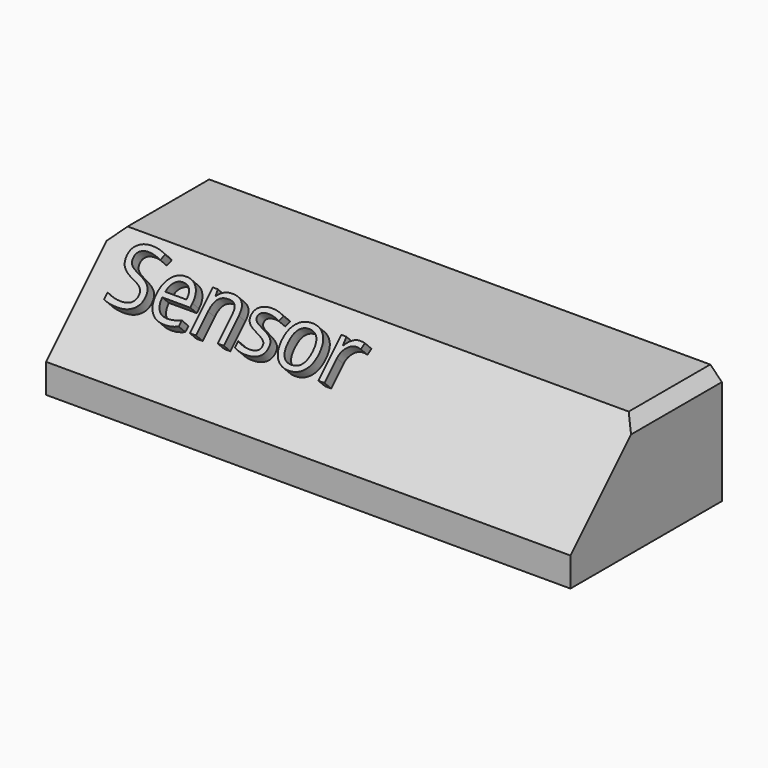
from build123d import *

# Parameters (mm, degrees)
F0_W         = 114.3
F0_H         = 41.275
F1_DEPTH     = 25.4
F2_SIZE      = 19.05
F3_SIZE      = 2.54
F4_TEXT_SIZE = 16.5284106818
F5_DEPTH     = 2.54


# Not quite as in the source:
# - Text() gives the source's letters only with a copy of the font that has no kerning and outlines rounded to 1/6400 em; it was checked with that copy


with BuildPart() as f1:
    # F0 (on Top) → F1 (new body)
    with BuildSketch(Plane.XY):
        with Locations((0, -20.6375)):
            Rectangle(F0_W, F0_H)
    extrude(amount=F1_DEPTH)

    # F2
    f2_edges = [f1.edges().sort_by_distance(p)[0] for p in [
        (0, -41.275, 25.4),
    ]]
    chamfer(f2_edges, length=F2_SIZE)

    # F3
    f3_edges = [f1.edges().sort_by_distance(p)[0] for p in [
        (57.15, -11.1125, 25.4),
        (-57.15, -11.1125, 25.4),
    ]]
    chamfer(f3_edges, length=F3_SIZE)

    # F4 (on face) → F5 (join)
    with BuildSketch(Plane(origin=(0, -23.8125, 23.8125), x_dir=(1, 0, 0), z_dir=(0, -0.7071067812, 0.7071067812))):
        with Locations((-51.3733290136, -11.9004556909)):
            Text('Sensor', F4_TEXT_SIZE, font='Open Sans', text_align=(TextAlign.LEFT, TextAlign.BOTTOM))
    extrude(amount=F5_DEPTH)


solid = f1.part
